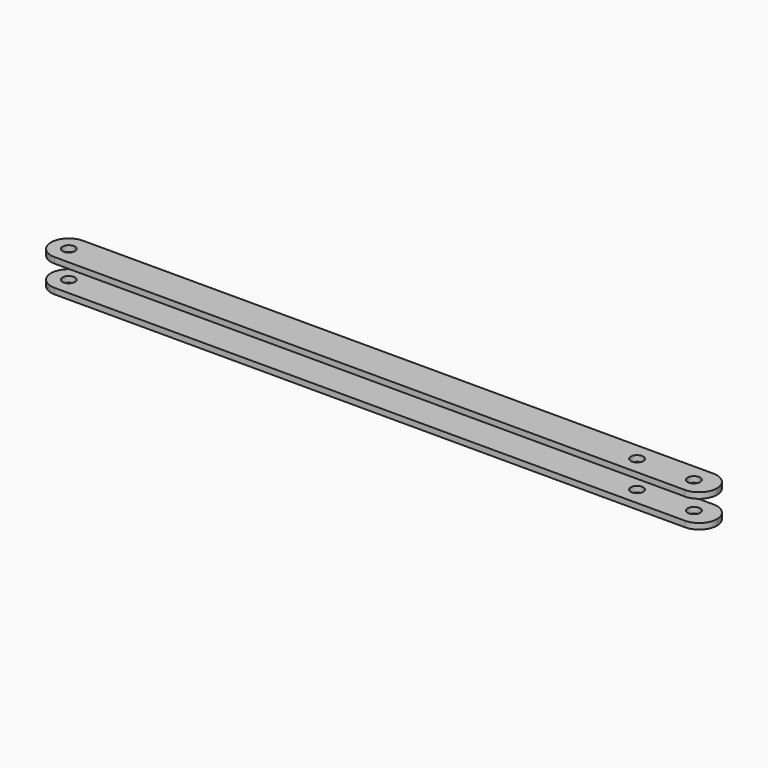
from build123d import *

# Parameters (mm, degrees)
F0_W     = 375
F0_H     = 3.2608695652
F1_DEPTH = 20
F2_R     = 9.99999
F2_2_R   = 9.99999
F3_R     = 3.5
F4_DEPTH = 25


# Not quite as in the source:
# - a fillet or chamfer is up to 0.001 mm smaller than in the source, because OpenCascade refuses the exact size
# - a feature names something its author has since deleted; it is built from what else it names


with BuildPart() as f1:
    # F0 (on Front) → F1 (new body)
    with BuildSketch(Plane.XZ):
        with Locations((143.1633904347, -7.0869565217)):
            Rectangle(F0_W, F0_H)
    extrude(amount=F1_DEPTH)

    # F2#2 (radius 10 in the source; OpenCascade refuses exactly that, so slightly less here)
    f2_2_edges = [f1.edges().sort_by_distance(p)[0] for p in [
        (330.66339, -20, -7.086957),
        (330.66339, 0, -7.086957),
        (-44.33661, 0, -7.086957),
        (-44.33661, -20, -7.086957),
    ]]
    fillet(f2_2_edges, radius=F2_2_R)


with BuildPart() as f1b:
    # F0 (on Front) → F1, piece 2 (new body)
    with BuildSketch(Plane.XZ):
        with Locations((143.1633904347, 8.1739130435)):
            Rectangle(F0_W, F0_H)
    extrude(amount=F1_DEPTH)

    # F2 (radius 10 in the source; OpenCascade refuses exactly that, so slightly less here)
    f2_edges = [f1b.edges().sort_by_distance(p)[0] for p in [
        (330.66339, -20, 8.173913),
        (330.66339, 0, 8.173913),
        (-44.33661, 0, 8.173913),
        (-44.33661, -20, 8.173913),
    ]]
    fillet(f2_edges, radius=F2_R)


with BuildPart() as f4_tool:
    # F3 (on face) → F4 (new body)
    with BuildSketch(Plane.XY.offset(9.8043478261)):
        with Locations((317.6633904347, -10)):
            Circle(F3_R)
        with Locations((285.6633904347, -10)):
            Circle(F3_R)
        with Locations((-34.3366095653, -10)):
            Circle(F3_R)
    extrude(amount=-F4_DEPTH)


with BuildPart() as f1_1:
    add(f1.part)

    # F4: cut by f4_tool
    add(f4_tool.part, mode=Mode.SUBTRACT)


with BuildPart() as f1b_1:
    add(f1b.part)

    # F4: cut by f4_tool
    add(f4_tool.part, mode=Mode.SUBTRACT)


solid = Compound([f1_1.part, f1b_1.part])
